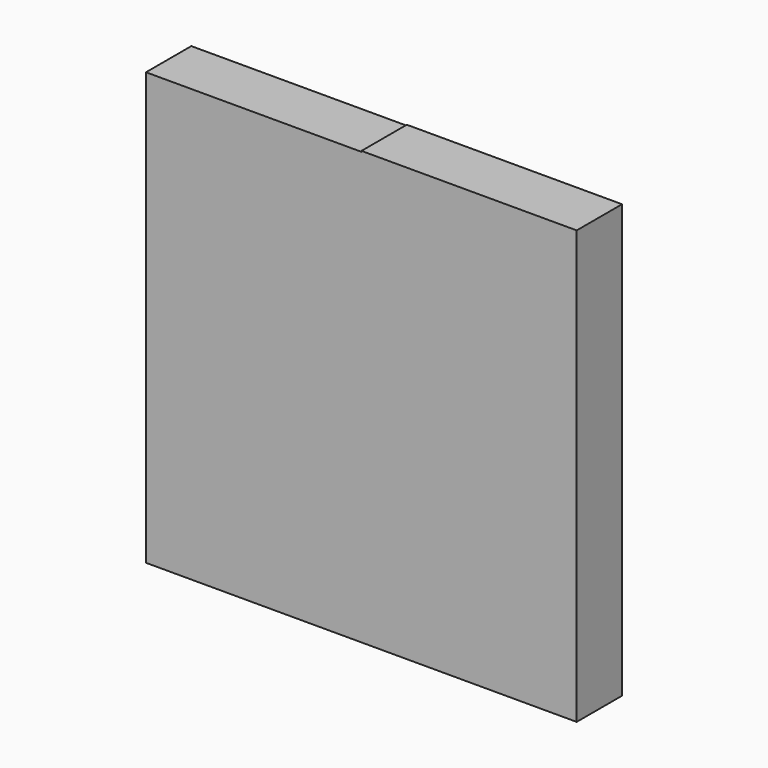
from build123d import *

# Parameters (mm, degrees)
F0_W     = 96.6067910194
F0_H     = 96.1308255792
F0_W_2   = 96.4857041836
F0_H_2   = 0.4863366485
F0_H_3   = 96.9959124923
F1_DEPTH = 25.4


with BuildPart() as f1:
    # F0 (on Front) → F1 (new body)
    with BuildSketch(Plane.XZ):
        Polygon((0, -0.4863366485), (0, 0), (-96.6067910194, 0), (-96.6067910194, -97.4822491407), (0, -97.4822491407), align=None)
        with Locations((-48.3033955097, 48.0654127896)):
            Rectangle(F0_W, F0_H)
        with Locations((48.2428520918, -0.2431683242)):
            Rectangle(F0_W_2, F0_H_2)
        Polygon((0, 96.1308255792), (0, 0), (96.4857041836, 0), (96.4857041836, 96.5095758438), (0, 96.5095758438), align=None)
        with Locations((48.2428520918, -48.9842928946)):
            Rectangle(F0_W_2, F0_H_3)
    extrude(amount=F1_DEPTH)


solid = f1.part
